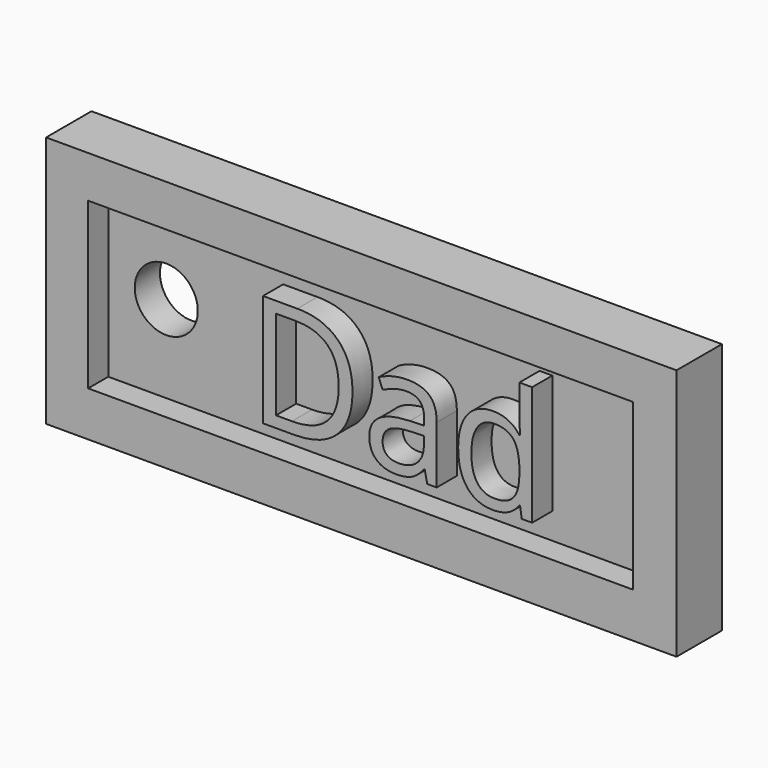
from build123d import *

# Parameters (mm, degrees)
F0_W         = 63.5
F0_H         = 25.4
F1_DEPTH     = 3.175
F2_W         = 63.5
F2_H         = 25.4
F2_W_2       = 54.8973740079
F2_H_2       = 16.6444173083
F3_DEPTH     = 2.54
F4_TEXT_SIZE = 15.8170639123
F5_DEPTH     = 2.54
F7_D         = 6.35


# Not quite as in the source:
# - Text() gives the source's letters only with a copy of the font that has no kerning and outlines rounded to 1/6400 em; it was checked with that copy


with BuildPart() as f1:
    # F0 (on Front) → F1 (new body)
    with BuildSketch(Plane.XZ):
        with Locations((31.75, 12.7)):
            Rectangle(F0_W, F0_H)
    extrude(amount=F1_DEPTH)

    # F2 (on face) → F3 (join)
    with BuildSketch(Plane.XZ.offset(3.175)):
        with Locations((31.75, 12.7)):
            Rectangle(F2_W, F2_H)
        with Locations((31.6827937495, 12.8483218141)):
            Rectangle(F2_W_2, F2_H_2, mode=Mode.SUBTRACT)
    extrude(amount=F3_DEPTH)

    # F4 (on face) → F5 (join)
    with BuildSketch(Plane.XZ.offset(3.175)):
        with Locations((20.2945079654, 7.1541788056)):
            Text('Dad', F4_TEXT_SIZE, font='Open Sans', text_align=(TextAlign.LEFT, TextAlign.BOTTOM))
    extrude(amount=F5_DEPTH)

    # F7 (through all)
    with Locations(Plane.XZ.offset(3.175)):
        with Locations((10.0742513314, 13.2863316685)):
            Hole(F7_D / 2)


solid = f1.part
